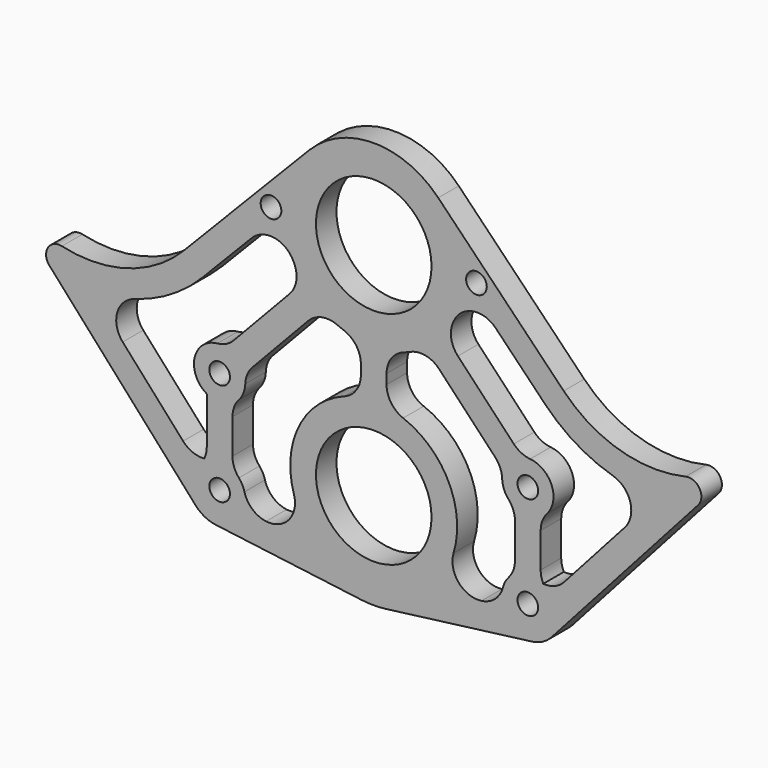
from build123d import *

# Parameters (mm, degrees)
F0_R        = 2.5527
F0_R_2      = 14.2875
F1_DEPTH    = 6.35
F3_DEPTH    = 25.4
F4_T1_DEPTH = 6.35


# Not quite as in the source:
# - a fillet or chamfer that OpenCascade refuses, or shapes differently, is made with other operations: its cross-section is extruded or revolved along the edge and cut away or added


with BuildPart() as f1:
    # F0 (on Front) → F1 (new body)
    with BuildSketch(Plane.XZ):
        with BuildLine():
            ThreePointArc((-3.0331353108, -25.2060360773), (0, -25.4), (3.0331353108, -25.2060360773))
            Line((3.0331353108, -25.2060360773), (39.1110451036, -20.5728453591))
            ThreePointArc((39.1110451036, -20.5728453591), (41.7972497423, -19.7238344651), (44.0177169487, -17.9900408661))
            Line((44.0177169487, -17.9900408661), (80.2059498117, 22.4920129361))
            ThreePointArc((80.2059498117, 22.4920129361), (80.5691803237, 26.2285207166), (77.1152341344, 27.6994668475))
            ThreePointArc((77.1152341344, 27.6994668475), (60.8820938076, 28.1479627769), (46.9763621139, 36.5352519414))
            Line((46.9763621139, 36.5352519414), (15.9477554983, 68.5021550209))
            ThreePointArc((15.9477554983, 68.5021550209), (0, 75.2475), (-15.9477554983, 68.5021550209))
            Line((-15.9477554983, 68.5021550209), (-46.9763621139, 36.5352519414))
            ThreePointArc((-46.9763621139, 36.5352519414), (-60.8820938076, 28.1479627769), (-77.1152341344, 27.6994668475))
            ThreePointArc((-77.1152341344, 27.6994668475), (-80.5691803237, 26.2285207166), (-80.2059498117, 22.4920129361))
            Line((-80.2059498117, 22.4920129361), (-44.0177169487, -17.9900408661))
            ThreePointArc((-44.0177169487, -17.9900408661), (-41.7972497423, -19.7238344651), (-39.1110451036, -20.5728453591))
            Line((-39.1110451036, -20.5728453591), (-3.0331353108, -25.2060360773))
        make_face()
        with Locations((-38.1, -12.7)):
            Circle(F0_R, mode=Mode.SUBTRACT)
        with Locations((0, -1.5875)):
            Circle(F0_R_2, mode=Mode.SUBTRACT)
        with Locations((-38.1, 12.7)):
            Circle(F0_R, mode=Mode.SUBTRACT)
        with Locations((38.1, -12.7)):
            Circle(F0_R, mode=Mode.SUBTRACT)
        with Locations((38.1, 12.7)):
            Circle(F0_R, mode=Mode.SUBTRACT)
        with Locations((-25.4, 53.0225)):
            Circle(F0_R, mode=Mode.SUBTRACT)
        with Locations((0, 53.0225)):
            Circle(F0_R_2, mode=Mode.SUBTRACT)
        with Locations((25.4, 53.0225)):
            Circle(F0_R, mode=Mode.SUBTRACT)
    extrude(amount=F1_DEPTH)

    # F2 (on face) → F3 (cut)
    with BuildSketch(Plane.XZ.offset(6.35)):
        with BuildLine():
            ThreePointArc((-43.3811914248, -9.1741643352), (-42.441704222, -8.0661997833), (-41.275, -7.200738686))
            Line((-41.275, -7.200738686), (-41.275, 7.200738686))
            ThreePointArc((-41.275, 7.200738686), (-44.0004697722, 15.046690535), (-36.6309164423, 18.8777255929))
            Line((-36.6309164423, 18.8777255929), (-17.4151480361, 39.2144138227))
            ThreePointArc((-17.4151480361, 39.2144138227), (-20.0010259245, 43.331804103), (-21.6296875, 47.9129752029))
            ThreePointArc((-21.6296875, 47.9129752029), (-24.6257359251, 46.7198802953), (-27.8214787465, 47.1523261797))
            Line((-27.8214787465, 47.1523261797), (-42.4198605429, 32.112493364))
            ThreePointArc((-42.4198605429, 32.112493364), (-54.9895844041, 23.5171709652), (-69.9173374643, 20.510559308))
            Line((-69.9173374643, 20.510559308), (-43.3811914248, -9.1741643352))
        make_face()
        with BuildLine():
            Line((-34.925, 7.200738686), (-34.925, -7.200738686))
            ThreePointArc((-34.925, -7.200738686), (-32.0996562634, -10.6219299715), (-32.2039292281, -15.0577212415))
            Line((-32.2039292281, -15.0577212415), (-13.1332337576, -17.5068145995))
            ThreePointArc((-13.1332337576, -17.5068145995), (-19.9026130173, 3.870741597), (-3.175, 18.8043067186))
            Line((-3.175, 18.8043067186), (-3.175, 31.0254547439))
            ThreePointArc((-3.175, 31.0254547439), (-8.2134168725, 32.3708557972), (-12.799622514, 34.8532873451))
            Line((-12.799622514, 34.8532873451), (-32.0153909201, 14.5165991152))
            ThreePointArc((-32.0153909201, 14.5165991152), (-32.1995302278, 10.353309465), (-34.925, 7.200738686))
        make_face()
        with BuildLine():
            Line((41.275, 7.200738686), (41.275, -7.200738686))
            ThreePointArc((41.275, -7.200738686), (42.441704222, -8.0661997833), (43.3811914248, -9.1741643352))
            Line((43.3811914248, -9.1741643352), (69.9173374643, 20.510559308))
            ThreePointArc((69.9173374643, 20.510559308), (54.9895844041, 23.5171709652), (42.4198605429, 32.112493364))
            Line((42.4198605429, 32.112493364), (27.8214787465, 47.1523261797))
            ThreePointArc((27.8214787465, 47.1523261797), (24.6257359251, 46.7198802953), (21.6296875, 47.9129752029))
            ThreePointArc((21.6296875, 47.9129752029), (20.0010259245, 43.331804103), (17.4151480361, 39.2144138227))
            Line((17.4151480361, 39.2144138227), (36.6309164423, 18.8777255929))
            ThreePointArc((36.6309164423, 18.8777255929), (44.0004697722, 15.046690535), (41.275, 7.200738686))
        make_face()
        with BuildLine():
            Line((13.1332337576, -17.5068145995), (32.2039292281, -15.0577212415))
            ThreePointArc((32.2039292281, -15.0577212415), (32.0996562634, -10.6219299715), (34.925, -7.200738686))
            Line((34.925, -7.200738686), (34.925, 7.200738686))
            ThreePointArc((34.925, 7.200738686), (32.1995302278, 10.353309465), (32.0153909201, 14.5165991152))
            Line((32.0153909201, 14.5165991152), (12.799622514, 34.8532873451))
            ThreePointArc((12.799622514, 34.8532873451), (8.2134168725, 32.3708557972), (3.175, 31.0254547439))
            Line((3.175, 31.0254547439), (3.175, 18.8043067186))
            ThreePointArc((3.175, 18.8043067186), (19.9026130173, 3.870741597), (13.1332337576, -17.5068145995))
        make_face()
    extrude(amount=-F3_DEPTH, mode=Mode.SUBTRACT)

    # F4: fillet of radius 6.35 on 31 edges, made by hand

    # F4_s2 → F4_t1 (join)
    with BuildSketch(Plane.XZ):
        with BuildLine():
            ThreePointArc((-25.4999328069, 46.6732863925), (-28.0274278752, 46.1917334318), (-30.1563671847, 44.7468313623))
            Line((-30.1563671847, 44.7468313623), (-27.8214787465, 47.1523261797))
            ThreePointArc((-27.8214787465, 47.1523261797), (-26.6832571196, 46.8035168705), (-25.4999328069, 46.6732863925))
        make_face()
        with BuildLine():
            ThreePointArc((-19.9098958333, 43.1459280792), (-22.2094720123, 45.6940981456), (-25.49921875, 46.6732751938))
            ThreePointArc((-25.49921875, 46.6732751938), (-23.4626186853, 46.9752647936), (-21.6296875, 47.9129752029))
            ThreePointArc((-21.6296875, 47.9129752029), (-20.9061098832, 45.4802725735), (-19.9098958333, 43.1459280792))
        make_face()
        with BuildLine():
            ThreePointArc((-20.8104553969, 35.621046866), (-19.1395225651, 39.0861033883), (-19.775762937, 42.8800237117))
            ThreePointArc((-19.775762937, 42.8800237117), (-18.6855596309, 40.9891926291), (-17.4151480361, 39.2144138227))
            Line((-17.4151480361, 39.2144138227), (-20.8104553969, 35.621046866))
        make_face()
        with BuildLine():
            ThreePointArc((-3.175, 23.6632332814), (-4.3022626627, 20.0513757668), (-7.2838235294, 17.721884274))
            ThreePointArc((-7.2838235294, 17.721884274), (-5.2573431495, 18.3691216895), (-3.175, 18.8043067186))
            Line((-3.175, 18.8043067186), (-3.175, 23.6632332814))
        make_face()
        with BuildLine():
            ThreePointArc((-38.6770301176, 19.0237280336), (-36.4785224973, 19.6361610946), (-34.6385347131, 20.9863295896))
            Line((-34.6385347131, 20.9863295896), (-36.6309164423, 18.8777255929))
            ThreePointArc((-36.6309164423, 18.8777255929), (-37.6480387039, 19.0338954038), (-38.6770301176, 19.0237280336))
        make_face()
        with BuildLine():
            ThreePointArc((-41.275, -4.2997395874), (-41.6851188985, -6.5448036176), (-42.8625, -8.4998697937))
            ThreePointArc((-42.8625, -8.4998697937), (-42.1215559142, -7.7857769659), (-41.275, -7.200738686))
            Line((-41.275, -7.200738686), (-41.275, -4.2997395874))
        make_face()
        with BuildLine():
            ThreePointArc((-47.1299420033, -4.9806154768), (-43.9553595951, -6.9040823934), (-40.2478842222, -6.724291392))
            ThreePointArc((-40.2478842222, -6.724291392), (-42.0112990938, -7.6975766474), (-43.3811914248, -9.1741643352))
            Line((-43.3811914248, -9.1741643352), (-47.1299420033, -4.9806154768))
        make_face()
        with BuildLine():
            ThreePointArc((-59.1117617466, 22.0497122742), (-63.433674019, 17.6998895462), (-62.0621747984, 11.7233626833))
            Line((-62.0621747984, 11.7233626833), (-69.9173374643, 20.510559308))
            ThreePointArc((-69.9173374643, 20.510559308), (-64.4593340972, 20.8924970257), (-59.1117617466, 22.0497122742))
        make_face()
        with BuildLine():
            ThreePointArc((-34.925, -4.2997395874), (-34.5148811015, -6.5448036176), (-33.3375, -8.4998697937))
            ThreePointArc((-33.3375, -8.4998697937), (-34.0784440858, -7.7857769659), (-34.925, -7.200738686))
            Line((-34.925, -7.200738686), (-34.925, -4.2997395874))
        make_face()
        with BuildLine():
            ThreePointArc((-33.3375, 8.4998697937), (-34.5148811015, 6.5448036176), (-34.925, 4.2997395874))
            Line((-34.925, 4.2997395874), (-34.925, 7.200738686))
            ThreePointArc((-34.925, 7.200738686), (-34.0784440858, 7.7857769659), (-33.3375, 8.4998697937))
        make_face()
        with BuildLine():
            ThreePointArc((-30.0230091909, 16.625203112), (-31.2668035127, 14.7117022115), (-31.7537418344, 12.4820383172))
            ThreePointArc((-31.7537418344, 12.4820383172), (-31.8018673776, 13.5099539932), (-32.0153909201, 14.5165991152))
            Line((-32.0153909201, 14.5165991152), (-30.0230091909, 16.625203112))
        make_face()
        with BuildLine():
            ThreePointArc((-31.9580280848, -11.087957509), (-30.0075511004, -14.2460167198), (-26.6248922524, -15.7741913054))
            Line((-26.6248922524, -15.7741913054), (-32.2039292281, -15.0577212415))
            ThreePointArc((-32.2039292281, -15.0577212415), (-31.762147528, -13.092588898), (-31.9580280848, -11.087957509))
        make_face()
        with BuildLine():
            ThreePointArc((3.175, 23.6632332814), (4.3022626627, 20.0513757668), (7.2838235294, 17.721884274))
            ThreePointArc((7.2838235294, 17.721884274), (5.2573431495, 18.3691216895), (3.175, 18.8043067186))
            Line((3.175, 18.8043067186), (3.175, 23.6632332814))
        make_face()
        with BuildLine():
            ThreePointArc((-26.6174183984, -15.7751511113), (-20.9556247606, -13.572152955), (-19.7359747119, -7.620551336))
            ThreePointArc((-19.7359747119, -7.620551336), (-17.161898691, -13.0494212861), (-13.1332337576, -17.5068145995))
            Line((-13.1332337576, -17.5068145995), (-26.6174183984, -15.7751511113))
        make_face()
        with BuildLine():
            ThreePointArc((26.6248922524, -15.7741913054), (30.0075511004, -14.2460167198), (31.9580280848, -11.087957509))
            ThreePointArc((31.9580280848, -11.087957509), (31.762147528, -13.092588898), (32.2039292281, -15.0577212415))
            Line((32.2039292281, -15.0577212415), (26.6248922524, -15.7741913054))
        make_face()
        with BuildLine():
            ThreePointArc((33.3375, -8.4998697937), (34.5148811015, -6.5448036176), (34.925, -4.2997395874))
            Line((34.925, -4.2997395874), (34.925, -7.200738686))
            ThreePointArc((34.925, -7.200738686), (34.0784440858, -7.7857769659), (33.3375, -8.4998697937))
        make_face()
        with BuildLine():
            ThreePointArc((26.6174183984, -15.7751511113), (20.9556247606, -13.572152955), (19.7359747119, -7.620551336))
            ThreePointArc((19.7359747119, -7.620551336), (17.161898691, -13.0494212861), (13.1332337576, -17.5068145995))
            Line((13.1332337576, -17.5068145995), (26.6174183984, -15.7751511113))
        make_face()
        with BuildLine():
            ThreePointArc((34.6385347131, 20.9863295896), (36.4785224973, 19.6361610946), (38.6770301176, 19.0237280336))
            ThreePointArc((38.6770301176, 19.0237280336), (37.6480387039, 19.0338954038), (36.6309164423, 18.8777255929))
            Line((36.6309164423, 18.8777255929), (34.6385347131, 20.9863295896))
        make_face()
        with BuildLine():
            ThreePointArc((42.8625, 8.4998697937), (41.6851188985, 6.5448036176), (41.275, 4.2997395874))
            Line((41.275, 4.2997395874), (41.275, 7.200738686))
            ThreePointArc((41.275, 7.200738686), (42.1215559142, 7.7857769659), (42.8625, 8.4998697937))
        make_face()
        with BuildLine():
            ThreePointArc((19.775762937, 42.8800237117), (19.1395225651, 39.0861033883), (20.8104553969, 35.621046866))
            Line((20.8104553969, 35.621046866), (17.4151480361, 39.2144138227))
            ThreePointArc((17.4151480361, 39.2144138227), (18.6855596309, 40.9891926291), (19.775762937, 42.8800237117))
        make_face()
        with BuildLine():
            ThreePointArc((-9.0062033853, 32.7040619305), (-12.8300676147, 33.1244136714), (-16.1949298747, 31.2599203883))
            Line((-16.1949298747, 31.2599203883), (-12.799622514, 34.8532873451))
            ThreePointArc((-12.799622514, 34.8532873451), (-10.955742935, 33.685428822), (-9.0062033853, 32.7040619305))
        make_face()
        with BuildLine():
            ThreePointArc((7.4083333333, 32.0685690508), (4.3402467111, 29.7479058461), (3.175, 26.0817316368))
            Line((3.175, 26.0817316368), (3.175, 31.0254547439))
            ThreePointArc((3.175, 31.0254547439), (5.317307399, 31.442952576), (7.4083333333, 32.0685690508))
        make_face()
        with BuildLine():
            ThreePointArc((-3.175, 26.0817316368), (-4.3402467111, 29.7479058461), (-7.4083333333, 32.0685690508))
            ThreePointArc((-7.4083333333, 32.0685690508), (-5.317307399, 31.442952576), (-3.175, 31.0254547439))
            Line((-3.175, 31.0254547439), (-3.175, 26.0817316368))
        make_face()
        with BuildLine():
            ThreePointArc((16.1949298747, 31.2599203883), (12.8300676147, 33.1244136714), (9.0062033853, 32.7040619305))
            ThreePointArc((9.0062033853, 32.7040619305), (10.955742935, 33.685428822), (12.799622514, 34.8532873451))
            Line((12.799622514, 34.8532873451), (16.1949298747, 31.2599203883))
        make_face()
        with BuildLine():
            ThreePointArc((31.7537418344, 12.4820383172), (31.2668035127, 14.7117022115), (30.0230091909, 16.625203112))
            Line((30.0230091909, 16.625203112), (32.0153909201, 14.5165991152))
            ThreePointArc((32.0153909201, 14.5165991152), (31.8018673776, 13.5099539932), (31.7537418344, 12.4820383172))
        make_face()
        with BuildLine():
            ThreePointArc((34.925, 4.2997395874), (34.5148811015, 6.5448036176), (33.3375, 8.4998697937))
            ThreePointArc((33.3375, 8.4998697937), (34.0784440858, 7.7857769659), (34.925, 7.200738686))
            Line((34.925, 7.200738686), (34.925, 4.2997395874))
        make_face()
        with BuildLine():
            ThreePointArc((62.0621747984, 11.7233626833), (63.433674019, 17.6998895462), (59.1117617466, 22.0497122742))
            ThreePointArc((59.1117617466, 22.0497122742), (64.4593340972, 20.8924970257), (69.9173374643, 20.510559308))
            Line((69.9173374643, 20.510559308), (62.0621747984, 11.7233626833))
        make_face()
        with BuildLine():
            ThreePointArc((25.49921875, 46.6732751938), (22.2094720123, 45.6940981456), (19.9098958333, 43.1459280792))
            ThreePointArc((19.9098958333, 43.1459280792), (20.9061098832, 45.4802725735), (21.6296875, 47.9129752029))
            ThreePointArc((21.6296875, 47.9129752029), (23.4626186853, 46.9752647936), (25.49921875, 46.6732751938))
        make_face()
        with BuildLine():
            ThreePointArc((30.1563671847, 44.7468313623), (28.0274278752, 46.1917334318), (25.4999328069, 46.6732863925))
            ThreePointArc((25.4999328069, 46.6732863925), (26.6832571196, 46.8035168705), (27.8214787465, 47.1523261797))
            Line((27.8214787465, 47.1523261797), (30.1563671847, 44.7468313623))
        make_face()
        with BuildLine():
            ThreePointArc((41.275, -4.2997395874), (41.6851188985, -6.5448036176), (42.8625, -8.4998697937))
            ThreePointArc((42.8625, -8.4998697937), (42.1215559142, -7.7857769659), (41.275, -7.200738686))
            Line((41.275, -7.200738686), (41.275, -4.2997395874))
        make_face()
        with BuildLine():
            ThreePointArc((40.2478842222, -6.724291392), (43.9553595951, -6.9040823934), (47.1299420033, -4.9806154768))
            Line((47.1299420033, -4.9806154768), (43.3811914248, -9.1741643352))
            ThreePointArc((43.3811914248, -9.1741643352), (42.0112990938, -7.6975766474), (40.2478842222, -6.724291392))
        make_face()
    extrude(amount=F4_T1_DEPTH)


solid = f1.part
